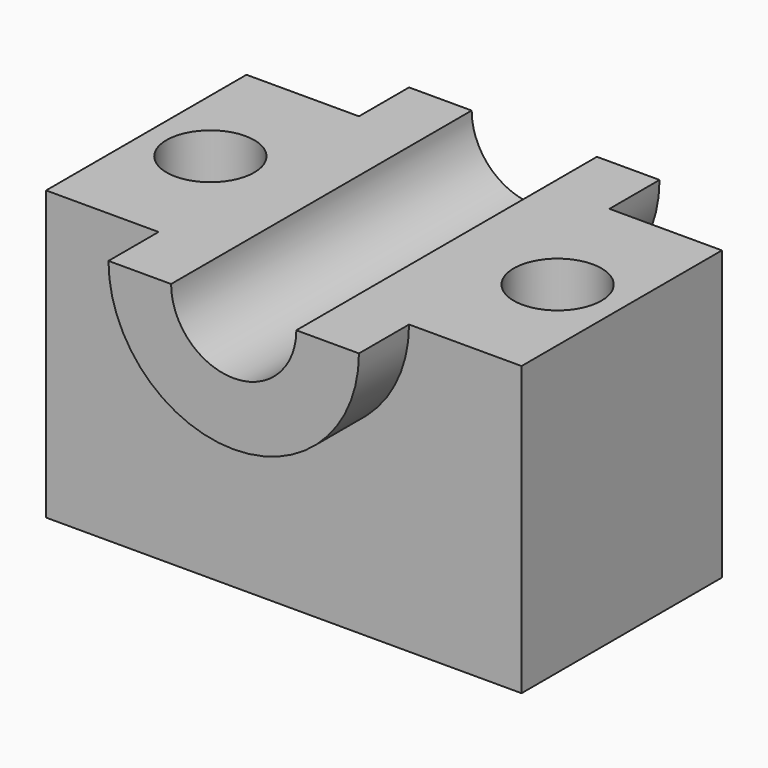
from build123d import *

# Parameters (mm, degrees)
F0_W     = 96.4296718666
F0_H     = 58.42
F1_DEPTH = 25.4
F4_DEPTH = 254
F6_DEPTH = 12.7
F2_R     = 8.8980244031
F7_DEPTH = 254


# Not quite as in the source:
# - a pattern or mirror of a feature is missing from the dataset's text; its kind, count and spacing are read off the source's solid


with BuildPart() as f1:
    # F0 (on Front) → F1 (new body, symmetric)
    with BuildSketch(Plane.XZ):
        Rectangle(F0_W, F0_H)
    extrude(amount=F1_DEPTH, both=True)

    # F3 (on face) → F4 (cut)
    with BuildSketch(Plane.XZ.offset(25.4)):
        with BuildLine():
            Line((12.7, 29.21), (-12.7, 29.21))
            ThreePointArc((-12.7, 29.21), (0, 16.51), (12.7, 29.21))
        make_face()
    extrude(amount=-F4_DEPTH, mode=Mode.SUBTRACT)

    # F5 (on face) → F6 (join)
    with BuildSketch(Plane(origin=(0, 25.4, 0), x_dir=(-1, 0, 0), z_dir=(0, 1, 0))):
        with BuildLine():
            Line((-12.7, 29.21), (-25.4, 29.21))
            ThreePointArc((-25.4, 29.21), (0, 3.81), (25.4, 29.21))
            Line((25.4, 29.21), (12.7, 29.21))
            ThreePointArc((12.7, 29.21), (0, 16.51), (-12.7, 29.21))
        make_face()
    f6 = extrude(amount=F6_DEPTH)

    # F6_copies: F6 across plane
    add(f6.mirror(Plane(origin=(0, 0, 0), x_dir=(0, 0, -1), z_dir=(0, -1, 0))))

    # F2 (on face) → F7 (cut)
    with BuildSketch(Plane.XY.offset(29.21)):
        with Locations((35.2072529495, 0)):
            Circle(F2_R)
        with Locations((-35.2072529495, 0)):
            Circle(F2_R)
    extrude(amount=-F7_DEPTH, mode=Mode.SUBTRACT)


solid = f1.part
